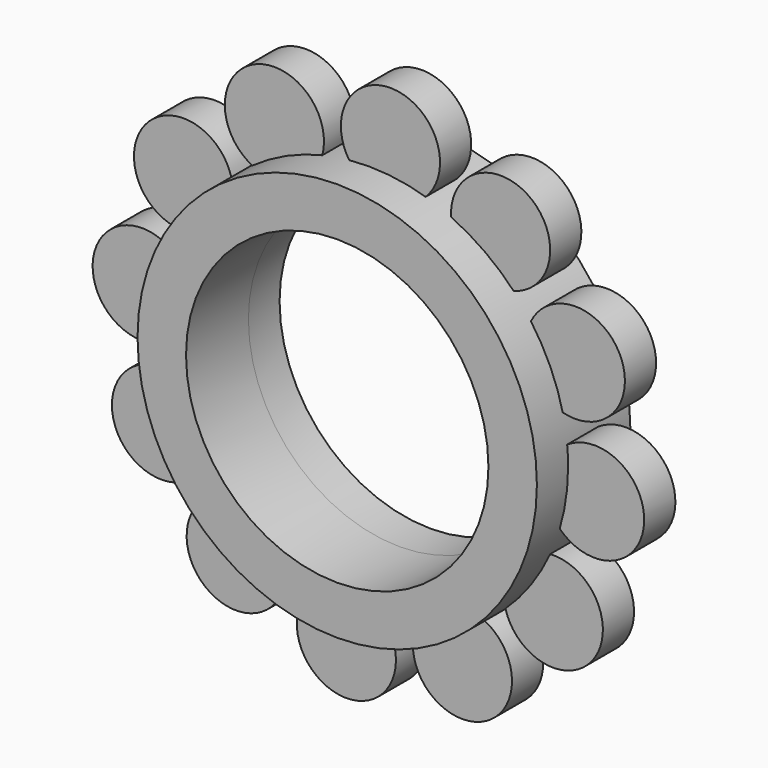
from build123d import *

# Parameters (mm, degrees)
F3_DEPTH      = 6.35
F4_R          = 32.5275336584
F4_R_2        = 24.6309625536
F5_DEPTH      = 12.7
F5_DEPTH_BACK = 6.35


# Not quite as in the source:
# - the program builds the solid bodies; features that only make, move or delete a surface that nothing else refers to are left out


with BuildPart() as f3:
    # F2 (on Front) → F3 (new body)
    with BuildSketch(Plane.XZ):
        with BuildLine():
            ThreePointArc((-57.3315931421, 32.0275125267), (-71.0548866609, 27.0779234756), (-58.5454572214, 19.5718331568))
            ThreePointArc((-58.5454572214, 19.5718331568), (-58.5431990279, 25.8586011297), (-57.3315931421, 32.0275125267))
        make_face()
    extrude(amount=F3_DEPTH)


with BuildPart() as f3b:
    # F2 (on Front) → F3, piece 2 (new body)
    with BuildSketch(Plane.XZ):
        with BuildLine():
            ThreePointArc((-48.4946400668, 46.3596213521), (-62.8541554032, 48.934798255), (-55.7737168812, 36.179618636))
            ThreePointArc((-55.7737168812, 36.179618636), (-52.6283772418, 41.6229903116), (-48.4946400668, 46.3596213521))
        make_face()
    extrude(amount=F3_DEPTH)


with BuildPart() as f3c:
    # F2 (on Front) → F3, piece 3 (new body)
    with BuildSketch(Plane.XZ):
        with BuildLine():
            ThreePointArc((-33.6755597989, 54.3531151471), (-44.8236764147, 63.7630414325), (-45.0694265942, 49.1765125916))
            ThreePointArc((-45.0694265942, 49.1765125916), (-39.6237967252, 52.3179409251), (-33.6755597989, 54.3531151471))
        make_face()
    extrude(amount=F3_DEPTH)


with BuildPart() as f3d:
    # F2 (on Front) → F3, piece 4 (new body)
    with BuildSketch(Plane.XZ):
        with BuildLine():
            ThreePointArc((-16.8451129286, 53.8661437046), (-21.7947019796, 67.5894372234), (-29.3007922985, 55.0800077839))
            ThreePointArc((-29.3007922985, 55.0800077839), (-23.0140243255, 55.0777495904), (-16.8451129286, 53.8661437046))
        make_face()
    extrude(amount=F3_DEPTH)


with BuildPart() as f3e:
    # F2 (on Front) → F3, piece 5 (new body)
    with BuildSketch(Plane.XZ):
        with BuildLine():
            ThreePointArc((-2.5130041032, 45.0291906293), (0.0621727998, 59.3887059657), (-12.6930068192, 52.3082674437))
            ThreePointArc((-12.6930068192, 52.3082674437), (-7.2496351437, 49.1629278043), (-2.5130041032, 45.0291906293))
        make_face()
    extrude(amount=F3_DEPTH)


with BuildPart() as f3f:
    # F2 (on Front) → F3, piece 6 (new body)
    with BuildSketch(Plane.XZ):
        with BuildLine():
            ThreePointArc((5.4804896918, 30.2101103614), (14.8904159772, 41.3582269772), (0.3038871363, 41.6039771567))
            ThreePointArc((0.3038871363, 41.6039771567), (3.4453154699, 36.1583472877), (5.4804896918, 30.2101103614))
        make_face()
    extrude(amount=F3_DEPTH)


with BuildPart() as f3g:
    # F2 (on Front) → F3, piece 7 (new body)
    with BuildSketch(Plane.XZ):
        with BuildLine():
            ThreePointArc((6.3584962121, 22.7035880089), (6.0154427046, 17.9919340198), (4.9935182493, 13.3796634911))
            ThreePointArc((4.9935182493, 13.3796634911), (18.7168117681, 18.3292525421), (6.2073823286, 25.835342861))
            ThreePointArc((6.2073823286, 25.835342861), (6.3206957771, 24.2712872673), (6.3584962121, 22.7035880089))
        make_face()
    extrude(amount=F3_DEPTH)


with BuildPart() as f3h:
    # F2 (on Front) → F3, piece 8 (new body)
    with BuildSketch(Plane.XZ):
        with BuildLine():
            ThreePointArc((3.4356419884, 9.2275573817), (0.290302349, 3.7841857062), (-3.843434826, -0.9524453343))
            ThreePointArc((-3.843434826, -0.9524453343), (10.5160805105, -3.5276222373), (3.4356419884, 9.2275573817))
        make_face()
    extrude(amount=F3_DEPTH)


with BuildPart() as f3i:
    # F2 (on Front) → F3, piece 9 (new body)
    with BuildSketch(Plane.XZ):
        with BuildLine():
            ThreePointArc((-23.0372825943, -9.6728317661), (-29.3240505672, -9.6705735727), (-35.4929619642, -8.4589676868))
            ThreePointArc((-35.4929619642, -8.4589676868), (-30.5433729131, -22.1822612056), (-23.0372825943, -9.6728317661))
        make_face()
    extrude(amount=F3_DEPTH)


with BuildPart() as f3j:
    # F2 (on Front) → F3, piece 10 (new body)
    with BuildSketch(Plane.XZ):
        with BuildLine():
            ThreePointArc((-7.2686482985, -3.7693365738), (-12.7142781676, -6.9107649074), (-18.6625150939, -8.9459391293))
            ThreePointArc((-18.6625150939, -8.9459391293), (-7.514398478, -18.3558654147), (-7.2686482985, -3.7693365738))
        make_face()
    extrude(amount=F3_DEPTH)


with BuildPart() as f3k:
    # F2 (on Front) → F3, piece 11 (new body)
    with BuildSketch(Plane.XZ):
        with BuildLine():
            ThreePointArc((-39.6450680735, -6.9010914259), (-45.0884397491, -3.7557517865), (-49.8250707896, 0.3779853885))
            ThreePointArc((-49.8250707896, 0.3779853885), (-52.4002476925, -13.981529948), (-39.6450680735, -6.9010914259))
        make_face()
    extrude(amount=F3_DEPTH)


with BuildPart() as f3l:
    # F2 (on Front) → F3, piece 12 (new body)
    with BuildSketch(Plane.XZ):
        with BuildLine():
            ThreePointArc((-52.6419620291, 3.803198861), (-55.7833903626, 9.2488287301), (-57.8185645846, 15.1970656564))
            ThreePointArc((-57.8185645846, 15.1970656564), (-67.22849087, 4.0489490405), (-52.6419620291, 3.803198861))
        make_face()
    extrude(amount=F3_DEPTH)


with BuildPart() as f5:
    # F4 (on Front) → F5 (new body, two sides)
    with BuildSketch(Plane.XZ) as f5_sk:
        with Locations((-26.1690374464, 22.7035880089)):
            Circle(F4_R)
        with Locations((-26.1690374464, 22.7035880089)):
            Circle(F4_R_2, mode=Mode.SUBTRACT)
    extrude(amount=F5_DEPTH)
    extrude(f5_sk.sketch, amount=-F5_DEPTH_BACK)


solid = Compound([f3.part, f3b.part, f3c.part, f3d.part, f3e.part, f3f.part, f3g.part, f3h.part, f3i.part, f3j.part, f3k.part, f3l.part, f5.part])
